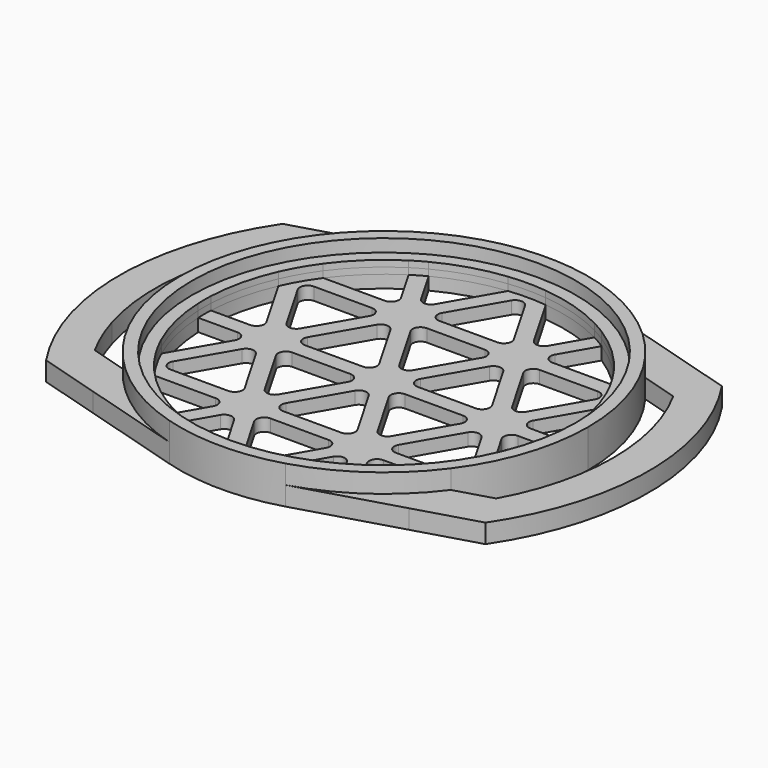
from build123d import *
from build123d import SkipClean  # not in build123d's __all__

# Parameters (mm, degrees)
F0_R     = 38.575
F1_DEPTH = 7.62
F2_DEPTH = 5.08
F3_DEPTH = 3.81
F4_R     = 36.075
F5_DEPTH = 1.27


with BuildPart() as f1:
    # F0 (on Top) → F1 (new body)
    with BuildSketch(Plane.XY):
        with BuildLine():
            ThreePointArc((32.9400932608, -24.4120924128), (38.9329155323, -12.8541078319), (41, 0))
            ThreePointArc((41, 0), (38.9329155323, 12.8541078319), (32.9400932608, 24.4120924128))
            ThreePointArc((32.9400932608, 24.4120924128), (23.5079959638, 33.5912805021), (11.6534709563, 39.3089889805))
            ThreePointArc((11.6534709563, 39.3089889805), (0, 41), (-11.6534709563, 39.3089889805))
            ThreePointArc((-11.6534709563, 39.3089889805), (-23.5079959638, 33.5912805021), (-32.9400932608, 24.4120924128))
            ThreePointArc((-32.9400932608, 24.4120924128), (-41, 0), (-32.9400932608, -24.4120924128))
            ThreePointArc((-32.9400932608, -24.4120924128), (-23.5079959638, -33.5912805021), (-11.6534709563, -39.3089889805))
            ThreePointArc((-11.6534709563, -39.3089889805), (0, -41), (11.6534709563, -39.3089889805))
            ThreePointArc((11.6534709563, -39.3089889805), (23.5079959638, -33.5912805021), (32.9400932608, -24.4120924128))
        make_face()
        Circle(F0_R, mode=Mode.SUBTRACT)
    extrude(amount=F1_DEPTH)

    # F0 (on Top) → F2 (join)
    with BuildSketch(Plane.XY):
        Circle(F0_R)
        with BuildLine():
            ThreePointArc((36.040053673, 1.5875), (36.0662623601, 0.7939422989), (36.075, 0))
            ThreePointArc((36.075, 0), (36.0662623601, -0.7939422989), (36.040053673, -1.5875))
            ThreePointArc((36.040053673, -1.5875), (35.1142128869, -8.2702888905), (32.9602474654, -14.6638232401))
            ThreePointArc((32.9602474654, -14.6638232401), (31.2418664415, -18.0375), (29.1793671753, -21.2125))
            ThreePointArc((29.1793671753, -21.2125), (24.7193867193, -26.2746559487), (19.394842165, -30.4178520345))
            ThreePointArc((19.394842165, -30.4178520345), (18.0375, -31.2418664415), (16.645211508, -32.0053520345))
            ThreePointArc((16.645211508, -32.0053520345), (10.3948261676, -34.5449448392), (3.7808802901, -35.8763232401))
            ThreePointArc((3.7808802901, -35.8763232401), (0, -36.075), (-3.7808802901, -35.8763232401))
            ThreePointArc((-3.7808802901, -35.8763232401), (-10.3948261676, -34.5449448392), (-16.645211508, -32.0053520345))
            ThreePointArc((-16.645211508, -32.0053520345), (-18.0375, -31.2418664415), (-19.394842165, -30.4178520345))
            ThreePointArc((-19.394842165, -30.4178520345), (-24.7193867193, -26.2746559487), (-29.1793671753, -21.2125))
            ThreePointArc((-29.1793671753, -21.2125), (-31.2418664415, -18.0375), (-32.9602474654, -14.6638232401))
            ThreePointArc((-32.9602474654, -14.6638232401), (-35.1142128869, -8.2702888905), (-36.040053673, -1.5875))
            ThreePointArc((-36.040053673, -1.5875), (-36.075, 0), (-36.040053673, 1.5875))
            ThreePointArc((-36.040053673, 1.5875), (-35.1142128869, 8.2702888905), (-32.9602474654, 14.6638232401))
            ThreePointArc((-32.9602474654, 14.6638232401), (-31.2418664415, 18.0375), (-29.1793671753, 21.2125))
            ThreePointArc((-29.1793671753, 21.2125), (-24.7193867193, 26.2746559487), (-19.394842165, 30.4178520345))
            ThreePointArc((-19.394842165, 30.4178520345), (-18.0375, 31.2418664415), (-16.645211508, 32.0053520345))
            ThreePointArc((-16.645211508, 32.0053520345), (-10.3948261676, 34.5449448392), (-3.7808802901, 35.8763232401))
            ThreePointArc((-3.7808802901, 35.8763232401), (0, 36.075), (3.7808802901, 35.8763232401))
            ThreePointArc((3.7808802901, 35.8763232401), (10.3948261676, 34.5449448392), (16.645211508, 32.0053520345))
            ThreePointArc((16.645211508, 32.0053520345), (18.0375, 31.2418664415), (19.394842165, 30.4178520345))
            ThreePointArc((19.394842165, 30.4178520345), (24.7193867193, 26.2746559487), (29.1793671753, 21.2125))
            ThreePointArc((29.1793671753, 21.2125), (31.2418664415, 18.0375), (32.9602474654, 14.6638232401))
            ThreePointArc((32.9602474654, 14.6638232401), (35.1142128869, 8.2702888905), (36.040053673, 1.5875))
        make_face(mode=Mode.SUBTRACT)
    extrude(amount=F2_DEPTH)

    # F0 (on Top) → F3 (join)
    with BuildSketch(Plane.XY):
        with BuildLine():
            ThreePointArc((36.040053673, -1.5875), (36.0662623601, -0.7939422989), (36.075, 0))
            ThreePointArc((36.075, 0), (36.0662623601, 0.7939422989), (36.040053673, 1.5875))
            Line((36.040053673, 1.5875), (28.1602593797, 1.5875))
            ThreePointArc((28.1602593797, 1.5875), (26.7854440512, 2.38125), (26.7854440512, 3.96875))
            Line((26.7854440512, 3.96875), (32.9602474654, 14.6638232401))
            ThreePointArc((32.9602474654, 14.6638232401), (31.2418664415, 18.0375), (29.1793671753, 21.2125))
            Line((29.1793671753, 21.2125), (16.8297603469, 21.2125))
            ThreePointArc((16.8297603469, 21.2125), (15.4549450184, 22.00625), (15.4549450184, 23.59375))
            Line((15.4549450184, 23.59375), (19.394842165, 30.4178520345))
            ThreePointArc((19.394842165, 30.4178520345), (18.0375, 31.2418664415), (16.645211508, 32.0053520345))
            Line((16.645211508, 32.0053520345), (12.7053143614, 25.18125))
            ThreePointArc((12.7053143614, 25.18125), (11.3304990328, 24.3875), (9.9556837043, 25.18125))
            Line((9.9556837043, 25.18125), (3.7808802901, 35.8763232401))
            ThreePointArc((3.7808802901, 35.8763232401), (0, 36.075), (-3.7808802901, 35.8763232401))
            Line((-3.7808802901, 35.8763232401), (-9.9556837043, 25.18125))
            ThreePointArc((-9.9556837043, 25.18125), (-11.3304990328, 24.3875), (-12.7053143614, 25.18125))
            Line((-12.7053143614, 25.18125), (-16.645211508, 32.0053520345))
            ThreePointArc((-16.645211508, 32.0053520345), (-18.0375, 31.2418664415), (-19.394842165, 30.4178520345))
            Line((-19.394842165, 30.4178520345), (-15.4549450184, 23.59375))
            ThreePointArc((-15.4549450184, 23.59375), (-15.4549450184, 22.00625), (-16.8297603469, 21.2125))
            Line((-16.8297603469, 21.2125), (-29.1793671753, 21.2125))
            ThreePointArc((-29.1793671753, 21.2125), (-31.2418664415, 18.0375), (-32.9602474654, 14.6638232401))
            Line((-32.9602474654, 14.6638232401), (-26.7854440512, 3.96875))
            ThreePointArc((-26.7854440512, 3.96875), (-26.7854440512, 2.38125), (-28.1602593797, 1.5875))
            Line((-28.1602593797, 1.5875), (-36.040053673, 1.5875))
            ThreePointArc((-36.040053673, 1.5875), (-36.075, 0), (-36.040053673, -1.5875))
            Line((-36.040053673, -1.5875), (-28.1602593797, -1.5875))
            ThreePointArc((-28.1602593797, -1.5875), (-26.7854440512, -2.38125), (-26.7854440512, -3.96875))
            Line((-26.7854440512, -3.96875), (-32.9602474654, -14.6638232401))
            ThreePointArc((-32.9602474654, -14.6638232401), (-31.2418664415, -18.0375), (-29.1793671753, -21.2125))
            Line((-29.1793671753, -21.2125), (-16.8297603469, -21.2125))
            ThreePointArc((-16.8297603469, -21.2125), (-15.4549450184, -22.00625), (-15.4549450184, -23.59375))
            Line((-15.4549450184, -23.59375), (-19.394842165, -30.4178520345))
            ThreePointArc((-19.394842165, -30.4178520345), (-18.0375, -31.2418664415), (-16.645211508, -32.0053520345))
            Line((-16.645211508, -32.0053520345), (-12.7053143614, -25.18125))
            ThreePointArc((-12.7053143614, -25.18125), (-11.3304990328, -24.3875), (-9.9556837043, -25.18125))
            Line((-9.9556837043, -25.18125), (-3.7808802901, -35.8763232401))
            ThreePointArc((-3.7808802901, -35.8763232401), (0, -36.075), (3.7808802901, -35.8763232401))
            Line((3.7808802901, -35.8763232401), (9.9556837043, -25.18125))
            ThreePointArc((9.9556837043, -25.18125), (11.3304990328, -24.3875), (12.7053143614, -25.18125))
            Line((12.7053143614, -25.18125), (16.645211508, -32.0053520345))
            ThreePointArc((16.645211508, -32.0053520345), (18.0375, -31.2418664415), (19.394842165, -30.4178520345))
            Line((19.394842165, -30.4178520345), (15.4549450184, -23.59375))
            ThreePointArc((15.4549450184, -23.59375), (15.4549450184, -22.00625), (16.8297603469, -21.2125))
            Line((16.8297603469, -21.2125), (29.1793671753, -21.2125))
            ThreePointArc((29.1793671753, -21.2125), (31.2418664415, -18.0375), (32.9602474654, -14.6638232401))
            Line((32.9602474654, -14.6638232401), (26.7854440512, -3.96875))
            ThreePointArc((26.7854440512, -3.96875), (26.7854440512, -2.38125), (28.1602593797, -1.5875))
            Line((28.1602593797, -1.5875), (36.040053673, -1.5875))
        make_face()
        with BuildLine():
            Line((-16.8297603469, -18.0375), (-28.4922357845, -18.0375))
            ThreePointArc((-28.4922357845, -18.0375), (-29.867051113, -17.24375), (-29.867051113, -15.65625))
            Line((-29.867051113, -15.65625), (-24.0358133942, -5.55625))
            ThreePointArc((-24.0358133942, -5.55625), (-22.6609980657, -4.7625), (-21.2861827372, -5.55625))
            Line((-21.2861827372, -5.55625), (-15.4549450184, -15.65625))
            ThreePointArc((-15.4549450184, -15.65625), (-15.4549450184, -17.24375), (-16.8297603469, -18.0375))
        make_face(mode=Mode.SUBTRACT)
        with BuildLine():
            ThreePointArc((-9.9556837043, -14.06875), (-11.3304990328, -14.8625), (-12.7053143614, -14.06875))
            Line((-12.7053143614, -14.06875), (-18.5365520802, -3.96875))
            ThreePointArc((-18.5365520802, -3.96875), (-18.5365520802, -2.38125), (-17.1617367517, -1.5875))
            Line((-17.1617367517, -1.5875), (-5.499261314, -1.5875))
            ThreePointArc((-5.499261314, -1.5875), (-4.1244459855, -2.38125), (-4.1244459855, -3.96875))
            Line((-4.1244459855, -3.96875), (-9.9556837043, -14.06875))
        make_face(mode=Mode.SUBTRACT)
        with BuildLine():
            ThreePointArc((1.3748153285, -33.69375), (0, -34.4875), (-1.3748153285, -33.69375))
            Line((-1.3748153285, -33.69375), (-7.2060530473, -23.59375))
            ThreePointArc((-7.2060530473, -23.59375), (-7.2060530473, -22.00625), (-5.8312377188, -21.2125))
            Line((-5.8312377188, -21.2125), (5.8312377188, -21.2125))
            ThreePointArc((5.8312377188, -21.2125), (7.2060530473, -22.00625), (7.2060530473, -23.59375))
            Line((7.2060530473, -23.59375), (1.3748153285, -33.69375))
        make_face(mode=Mode.SUBTRACT)
        with BuildLine():
            Line((5.8312377188, -18.0375), (-5.8312377188, -18.0375))
            ThreePointArc((-5.8312377188, -18.0375), (-7.2060530473, -17.24375), (-7.2060530473, -15.65625))
            Line((-7.2060530473, -15.65625), (-1.3748153285, -5.55625))
            ThreePointArc((-1.3748153285, -5.55625), (0, -4.7625), (1.3748153285, -5.55625))
            Line((1.3748153285, -5.55625), (7.2060530473, -15.65625))
            ThreePointArc((7.2060530473, -15.65625), (7.2060530473, -17.24375), (5.8312377188, -18.0375))
        make_face(mode=Mode.SUBTRACT)
        with BuildLine():
            Line((24.0358133942, -5.55625), (29.867051113, -15.65625))
            ThreePointArc((29.867051113, -15.65625), (29.867051113, -17.24375), (28.4922357845, -18.0375))
            Line((28.4922357845, -18.0375), (16.8297603469, -18.0375))
            ThreePointArc((16.8297603469, -18.0375), (15.4549450184, -17.24375), (15.4549450184, -15.65625))
            Line((15.4549450184, -15.65625), (21.2861827372, -5.55625))
            ThreePointArc((21.2861827372, -5.55625), (22.6609980657, -4.7625), (24.0358133942, -5.55625))
        make_face(mode=Mode.SUBTRACT)
        with BuildLine():
            ThreePointArc((17.1617367517, -1.5875), (18.5365520802, -2.38125), (18.5365520802, -3.96875))
            Line((18.5365520802, -3.96875), (12.7053143614, -14.06875))
            ThreePointArc((12.7053143614, -14.06875), (11.3304990328, -14.8625), (9.9556837043, -14.06875))
            Line((9.9556837043, -14.06875), (4.1244459855, -3.96875))
            ThreePointArc((4.1244459855, -3.96875), (4.1244459855, -2.38125), (5.499261314, -1.5875))
            Line((5.499261314, -1.5875), (17.1617367517, -1.5875))
        make_face(mode=Mode.SUBTRACT)
        with BuildLine():
            Line((-18.5365520802, 3.96875), (-12.7053143614, 14.06875))
            ThreePointArc((-12.7053143614, 14.06875), (-11.3304990328, 14.8625), (-9.9556837043, 14.06875))
            Line((-9.9556837043, 14.06875), (-4.1244459855, 3.96875))
            ThreePointArc((-4.1244459855, 3.96875), (-4.1244459855, 2.38125), (-5.499261314, 1.5875))
            Line((-5.499261314, 1.5875), (-17.1617367517, 1.5875))
            ThreePointArc((-17.1617367517, 1.5875), (-18.5365520802, 2.38125), (-18.5365520802, 3.96875))
        make_face(mode=Mode.SUBTRACT)
        with BuildLine():
            ThreePointArc((-29.867051113, 15.65625), (-29.867051113, 17.24375), (-28.4922357845, 18.0375))
            Line((-28.4922357845, 18.0375), (-16.8297603469, 18.0375))
            ThreePointArc((-16.8297603469, 18.0375), (-15.4549450184, 17.24375), (-15.4549450184, 15.65625))
            Line((-15.4549450184, 15.65625), (-21.2861827372, 5.55625))
            ThreePointArc((-21.2861827372, 5.55625), (-22.6609980657, 4.7625), (-24.0358133942, 5.55625))
            Line((-24.0358133942, 5.55625), (-29.867051113, 15.65625))
        make_face(mode=Mode.SUBTRACT)
        with BuildLine():
            Line((12.7053143614, 14.06875), (18.5365520802, 3.96875))
            ThreePointArc((18.5365520802, 3.96875), (18.5365520802, 2.38125), (17.1617367517, 1.5875))
            Line((17.1617367517, 1.5875), (5.499261314, 1.5875))
            ThreePointArc((5.499261314, 1.5875), (4.1244459855, 2.38125), (4.1244459855, 3.96875))
            Line((4.1244459855, 3.96875), (9.9556837043, 14.06875))
            ThreePointArc((9.9556837043, 14.06875), (11.3304990328, 14.8625), (12.7053143614, 14.06875))
        make_face(mode=Mode.SUBTRACT)
        with BuildLine():
            ThreePointArc((-7.2060530473, 15.65625), (-7.2060530473, 17.24375), (-5.8312377188, 18.0375))
            Line((-5.8312377188, 18.0375), (5.8312377188, 18.0375))
            ThreePointArc((5.8312377188, 18.0375), (7.2060530473, 17.24375), (7.2060530473, 15.65625))
            Line((7.2060530473, 15.65625), (1.3748153285, 5.55625))
            ThreePointArc((1.3748153285, 5.55625), (0, 4.7625), (-1.3748153285, 5.55625))
            Line((-1.3748153285, 5.55625), (-7.2060530473, 15.65625))
        make_face(mode=Mode.SUBTRACT)
        with BuildLine():
            ThreePointArc((28.4922357845, 18.0375), (29.867051113, 17.24375), (29.867051113, 15.65625))
            Line((29.867051113, 15.65625), (24.0358133942, 5.55625))
            ThreePointArc((24.0358133942, 5.55625), (22.6609980657, 4.7625), (21.2861827372, 5.55625))
            Line((21.2861827372, 5.55625), (15.4549450184, 15.65625))
            ThreePointArc((15.4549450184, 15.65625), (15.4549450184, 17.24375), (16.8297603469, 18.0375))
            Line((16.8297603469, 18.0375), (28.4922357845, 18.0375))
        make_face(mode=Mode.SUBTRACT)
        with BuildLine():
            Line((-7.2060530473, 23.59375), (-1.3748153285, 33.69375))
            ThreePointArc((-1.3748153285, 33.69375), (0, 34.4875), (1.3748153285, 33.69375))
            Line((1.3748153285, 33.69375), (7.2060530473, 23.59375))
            ThreePointArc((7.2060530473, 23.59375), (7.2060530473, 22.00625), (5.8312377188, 21.2125))
            Line((5.8312377188, 21.2125), (-5.8312377188, 21.2125))
            ThreePointArc((-5.8312377188, 21.2125), (-7.2060530473, 22.00625), (-7.2060530473, 23.59375))
        make_face(mode=Mode.SUBTRACT)
        with BuildLine():
            ThreePointArc((-40.31749969, 22.225), (-36.4507899361, 28.1210120601), (-31.7290809885, 33.3574103593))
            Line((-31.7290809885, 33.3574103593), (-44.12749969, 29.6817978343))
            ThreePointArc((-44.12749969, 29.6817978343), (-53.18125, 0), (-44.12749969, -29.6817978343))
            Line((-44.12749969, -29.6817978343), (-31.7290809885, -33.3574103593))
            ThreePointArc((-31.7290809885, -33.3574103593), (-36.4507899361, -28.1210120601), (-40.31749969, -22.225))
            ThreePointArc((-40.31749969, -22.225), (-42.467054594, -17.7764079712), (-44.12749969, -13.1230780445))
            ThreePointArc((-44.12749969, -13.1230780445), (-46.0375, 0), (-44.12749969, 13.1230780445))
            ThreePointArc((-44.12749969, 13.1230780445), (-42.467054594, 17.7764079712), (-40.31749969, 22.225))
        make_face()
        with BuildLine():
            Line((-31.7290809885, -33.3574103593), (-11.6534709563, -39.3089889805))
            ThreePointArc((-11.6534709563, -39.3089889805), (-23.5079959638, -33.5912805021), (-32.9400932608, -24.4120924128))
            Line((-32.9400932608, -24.4120924128), (-40.31749969, -22.225))
            ThreePointArc((-40.31749969, -22.225), (-36.4507899361, -28.1210120601), (-31.7290809885, -33.3574103593))
        make_face()
        with BuildLine():
            ThreePointArc((-32.9400932608, 24.4120924128), (-23.5079959638, 33.5912805021), (-11.6534709563, 39.3089889805))
            Line((-11.6534709563, 39.3089889805), (-31.7290809885, 33.3574103593))
            ThreePointArc((-31.7290809885, 33.3574103593), (-36.4507899361, 28.1210120601), (-40.31749969, 22.225))
            Line((-40.31749969, 22.225), (-32.9400932608, 24.4120924128))
        make_face()
        with BuildLine():
            ThreePointArc((11.6534709563, 39.3089889805), (23.5079959638, 33.5912805021), (32.9400932608, 24.4120924128))
            Line((32.9400932608, 24.4120924128), (40.31749969, 22.225))
            ThreePointArc((40.31749969, 22.225), (36.4507899361, 28.1210120601), (31.7290809885, 33.3574103593))
            Line((31.7290809885, 33.3574103593), (11.6534709563, 39.3089889805))
        make_face()
        with BuildLine():
            ThreePointArc((31.7290809885, 33.3574103593), (36.4507899361, 28.1210120601), (40.31749969, 22.225))
            ThreePointArc((40.31749969, 22.225), (46.0375, 0), (40.31749969, -22.225))
            ThreePointArc((40.31749969, -22.225), (36.4507899361, -28.1210120601), (31.7290809885, -33.3574103593))
            Line((31.7290809885, -33.3574103593), (44.12749969, -29.6817978343))
            ThreePointArc((44.12749969, -29.6817978343), (53.18125, 0), (44.12749969, 29.6817978343))
            Line((44.12749969, 29.6817978343), (31.7290809885, 33.3574103593))
        make_face()
        with BuildLine():
            Line((40.31749969, -22.225), (32.9400932608, -24.4120924128))
            ThreePointArc((32.9400932608, -24.4120924128), (23.5079959638, -33.5912805021), (11.6534709563, -39.3089889805))
            Line((11.6534709563, -39.3089889805), (31.7290809885, -33.3574103593))
            ThreePointArc((31.7290809885, -33.3574103593), (36.4507899361, -28.1210120601), (40.31749969, -22.225))
        make_face()
    extrude(amount=F3_DEPTH)

    # F4 (on face) → F5 (cut)
    with BuildSketch(Plane.XY.offset(3.81)):
        Circle(F4_R)
    with SkipClean():  # cleaning this boolean's faces spoils the solid; the shape is the same uncleaned
        extrude(amount=-F5_DEPTH, mode=Mode.SUBTRACT)


solid = f1.part
